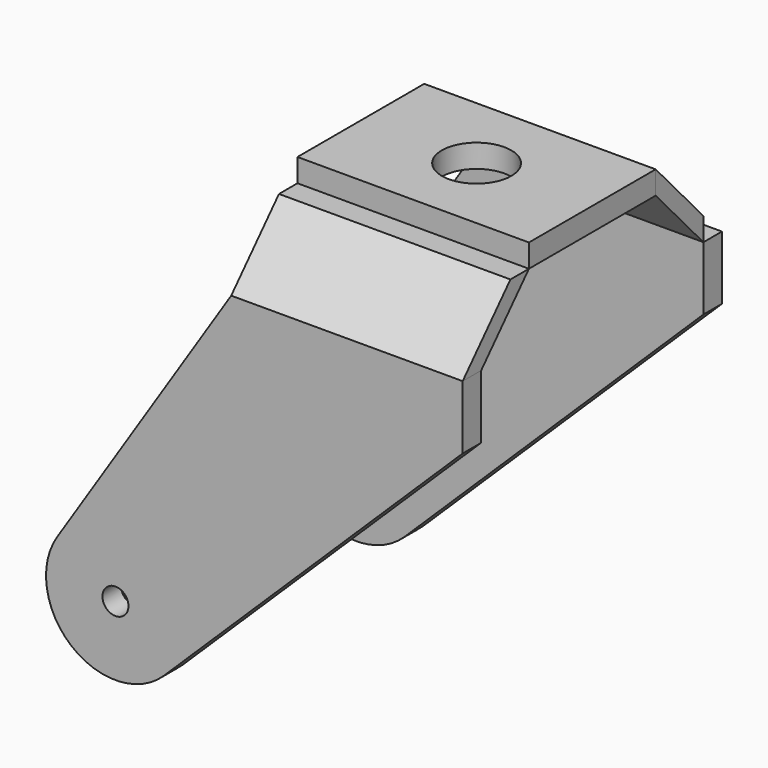
from build123d import *

# Parameters (mm, degrees)
F2_R      = 7.14375
F7_W      = 127
F7_H      = 48.524113
F10_DEPTH = 12.7
F5_W      = 127
F5_H      = 86.9188
F5_R      = 19.05
F9_W      = 127
F9_H      = 48.524112
F11_DEPTH = 12.7
F0_R      = 7.14375
F12_DEPTH = 12.7


with BuildPart() as f10:
    # F2 (on offset) + F7 (on 3pt) → F10 (new body)
    with BuildSketch(Plane.XZ.offset(152.4)):
        with BuildLine():
            Line((63.5, 168.275), (-31.987965, 20.697345))
            ThreePointArc((-31.987965, 20.697345), (-24.101451, -29.508135), (26.66774, -27.211057))
            Line((26.66774, -27.211057), (190.5, 133.35))
            Line((190.5, 133.35), (190.5, 168.275))
            Line((190.5, 168.275), (63.5, 168.275))
        make_face()
        Circle(F2_R, mode=Mode.SUBTRACT)
    with BuildSketch(Plane(origin=(0, -166.818574, 152.502937), x_dir=(-1, 0, 0), z_dir=(0, 0.738066, -0.674728))):
        with Locations((-127, 45.631502)):
            Rectangle(F7_W, F7_H)
    extrude(amount=F10_DEPTH, dir=(0, -1, 0))


with BuildPart() as f11:
    # F5 (on offset) + F9 (on 3pt) → F11 (new body)
    with BuildSketch(Plane.XY.offset(204.089)):
        with Locations((127, -76.2)):
            Rectangle(F5_W, F5_H)
        with Locations((127, -76.2)):
            Circle(F5_R, mode=Mode.SUBTRACT)
    with BuildSketch(Plane(origin=(0, 83.79997, 76.608625), x_dir=(1, 0, 0), z_dir=(0, -0.738066, -0.674728))):
        with Locations((127, 148.460121)):
            Rectangle(F9_W, F9_H)
    extrude(amount=F11_DEPTH, dir=(0, 0, 1))


with BuildPart() as f12:
    # F0 (on Front) → F12 (new body)
    with BuildSketch(Plane.XZ):
        with BuildLine():
            Line((63.5, 168.275), (-31.987965, 20.697345))
            ThreePointArc((-31.987965, 20.697345), (-24.101451, -29.508135), (26.66774, -27.211057))
            Line((26.66774, -27.211057), (190.5, 133.35))
            Line((190.5, 133.35), (190.5, 168.275))
            Line((190.5, 168.275), (63.5, 168.275))
        make_face()
        Circle(F0_R, mode=Mode.SUBTRACT)
    extrude(amount=-F12_DEPTH)


solid = Compound([f10.part, f11.part, f12.part])
